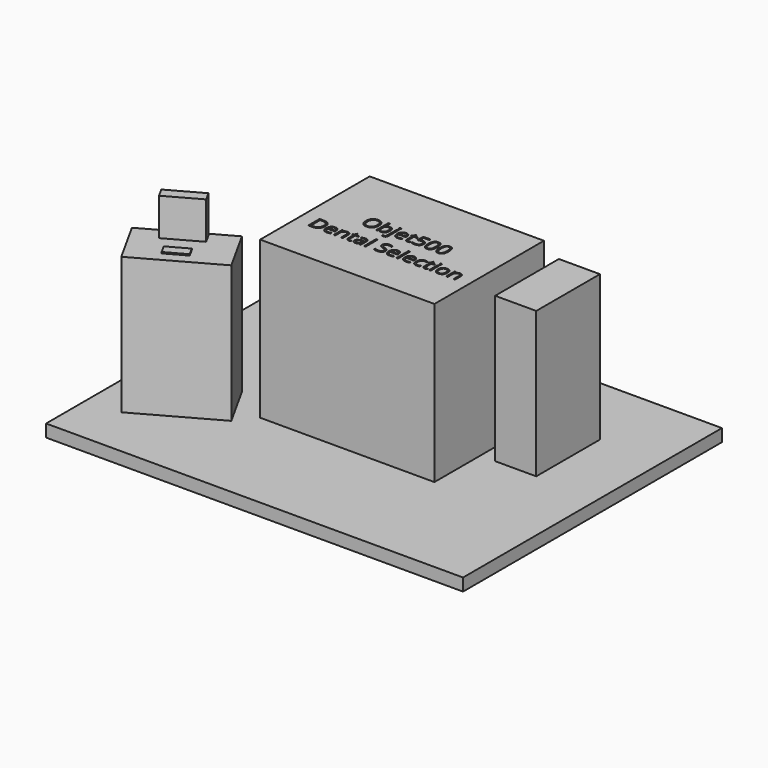
from build123d import *

# Parameters (mm, degrees)
F0_W          = 3350
F0_H          = 2600
F1_DEPTH      = 100
F2_W          = 1400
F2_H          = 1100
F3_DEPTH      = 1260
F4_W          = 330
F4_H          = 640
F5_DEPTH      = 1170
F6_W          = 845
F6_H          = 176.8575310707
F6_W_2        = 165
F7_DEPTH      = 300
F8_R          = 200
F10_DEPTH     = 439
F12_DEPTH     = 1100
F14_DEPTH     = 300
F15_DEPTH     = 300
F17_DEPTH     = 10
F18_TEXT_SIZE = 159.9652618585
F19_DEPTH     = 500


# Not quite as in the source:
# - Text() gives the source's letters only with a copy of the font that has no kerning and outlines rounded to 1/6400 em; it was checked with that copy


with BuildPart() as f1:
    # F0 (on Top) → F1 (new body)
    with BuildSketch(Plane.XY):
        Rectangle(F0_W, F0_H)
    extrude(amount=F1_DEPTH)

    # F2 (on face) → F3 (join)
    with BuildSketch(Plane.XY.offset(100)):
        with Locations((25, 150)):
            Rectangle(F2_W, F2_H)
    extrude(amount=F3_DEPTH)

    # F4 (on face) → F5 (join)
    with BuildSketch(Plane.XY.offset(100)):
        with Locations((1010, 380)):
            Rectangle(F4_W, F4_H)
    extrude(amount=F5_DEPTH)

    # F6 (on face) → F7 (join)
    with BuildSketch(Plane(origin=(0, 700, 0), x_dir=(-1, 0, 0), z_dir=(0, 1, 0))):
        with Locations((-422.5, 726.016074419)):
            Rectangle(F6_W, F6_H)
        with Locations((-927.5, 726.016074419)):
            Rectangle(F6_W_2, F6_H)
    extrude(amount=F7_DEPTH)

    # F8
    f8_edges = [f1.edges().sort_by_distance(p)[0] for p in [
        (1010, 1000, 726.016074),
        (0, 1000, 726.016074),
    ]]
    fillet(f8_edges, radius=F8_R)

    # F9 (on face) → F10 (cut)
    with BuildSketch(Plane.XY.offset(814.4448399544)):
        with BuildLine():
            Line((810, 900), (200, 900))
            ThreePointArc((200, 900), (129.2893218813, 870.7106781187), (100, 800))
            Line((100, 800), (100, 700))
            Line((100, 700), (725, 700))
            Line((725, 700), (845, 700))
            Line((845, 700), (910, 700))
            Line((910, 700), (910, 800))
            ThreePointArc((910, 800), (880.7106781187, 870.7106781187), (810, 900))
        make_face()
    extrude(amount=-F10_DEPTH, mode=Mode.SUBTRACT)

    # F11 (on face) → F12 (join)
    with BuildSketch(Plane.XY.offset(100)):
        Polygon((-983.9345267026, -196.9333749578), (-1595.8446390902, -536.8833923983), (-1401.5874862671, -886.5463137627), (-789.6773738795, -546.5962963222), align=None)
    extrude(amount=F12_DEPTH)

    # F13 (on face) → F14 (join)
    with BuildSketch(Plane.XY.offset(1200)):
        Polygon((-1154.086076436, -320.5210052314), (-1416.3332674593, -466.2138698488), (-1374.7628789658, -541.0405790415), (-1112.5156879425, -395.3477144241), align=None)
    extrude(amount=F14_DEPTH)

    # F13 (on face) → F15 (join)
    with BuildSketch(Plane.XY.offset(1200)):
        Polygon((-1154.086076436, -320.5210052314), (-1416.3332674593, -466.2138698488), (-1374.7628789658, -541.0405790415), (-1112.5156879425, -395.3477144241), align=None)
    extrude(amount=F15_DEPTH)

    # F16 (on face) → F17 (join)
    with BuildSketch(Plane.XY.offset(1200)):
        Polygon((-1113.8937216214, -538.1072461273), (-1269.9866666123, -624.8255374217), (-1232.2234010931, -692.7994243536), (-1076.1304561022, -606.0811330592), align=None)
    extrude(amount=F17_DEPTH)

    # F18 (on face) → F19 (cut)
    with BuildSketch(Plane.XY.offset(1360)):
        with Locations((-325.6041589337, 155.5693070107)):
            Text('Objet500', F18_TEXT_SIZE, font='Open Sans', text_align=(TextAlign.LEFT, TextAlign.BOTTOM))
        with Locations((-575, -61.9834491169)):
            Text('Dental Selection', F18_TEXT_SIZE, font='Open Sans', text_align=(TextAlign.LEFT, TextAlign.BOTTOM))
    extrude(amount=-F19_DEPTH, mode=Mode.SUBTRACT)


solid = f1.part
